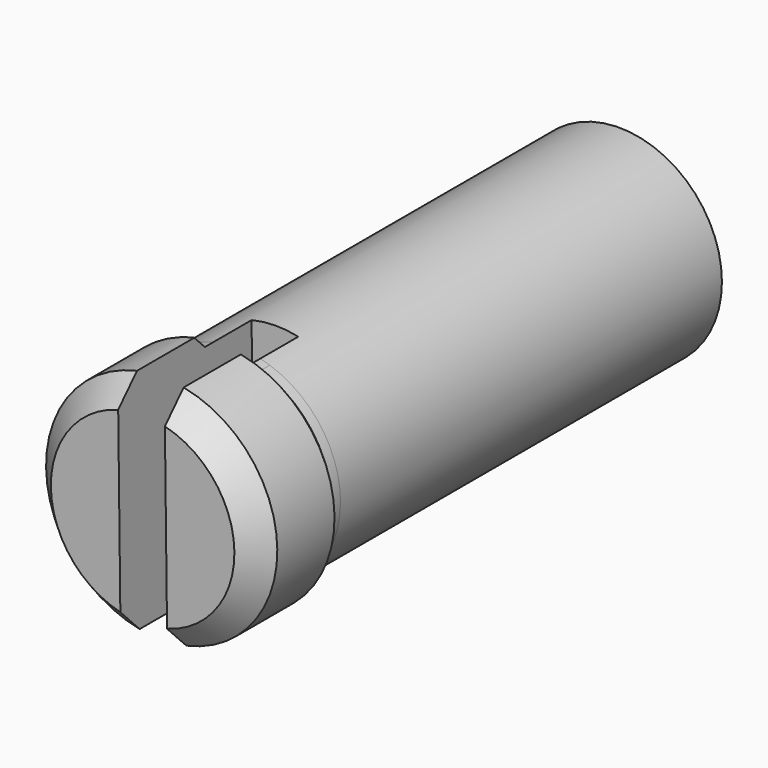
from build123d import *

# Parameters (mm, degrees)
F0_R         = 48.5
F0_R_2       = 43
F1_DEPTH     = 250
F2_DEPTH     = 200
F4_DEPTH     = 70
F5_T2_ANGLE  = 217.5315587112
F5_T4_ANGLE  = 217.5315587112
F5_T8_ANGLE  = 217.5315587112
F5_S9_R      = 43
F5_T10_DEPTH = 60
F5_T14_ANGLE = 217.5315587112
F5_S15_R     = 43
F5_T16_DEPTH = 60


# Not quite as in the source:
# - a fillet or chamfer that OpenCascade refuses, or shapes differently, is made with other operations: its cross-section is extruded or revolved along the edge and cut away or added


with BuildPart() as f1:
    # F0 (on Front) → F1 (new body)
    with BuildSketch(Plane.XZ):
        Circle(F0_R)
        Circle(F0_R_2, mode=Mode.SUBTRACT)
        Circle(F0_R_2)
    extrude(amount=F1_DEPTH)

    # F0 (on Front) → F2 (cut)
    with BuildSketch(Plane.XZ):
        Circle(F0_R)
        Circle(F0_R_2, mode=Mode.SUBTRACT)
    extrude(amount=F2_DEPTH, mode=Mode.SUBTRACT)

    # F3 (on face) → F4 (cut)
    with BuildSketch(Plane.XZ.offset(250)):
        with BuildLine():
            Line((10.3677597397, -47.3788935918), (9.2215594636, 47.6152584899))
            ThreePointArc((9.2215594636, 47.6152584899), (-0.5851588327, 48.4964698627), (-10.3677597397, 47.3788935918))
            Line((-10.3677597397, 47.3788935918), (-9.2215594636, -47.6152584899))
            ThreePointArc((-9.2215594636, -47.6152584899), (0.5851588327, -48.4964698627), (10.3677597397, -47.3788935918))
        make_face()
    extrude(amount=-F4_DEPTH, mode=Mode.SUBTRACT)

    # F5: chamfer of 10 on 4 edges, made by hand

    # F5_s1 → F5_t2 (revolve, cut)
    with BuildSketch(Plane(origin=(0, 0, 0), x_dir=(0, 1, 0), z_dir=(0.9506540069, 0, -0.3102530567))):
        Polygon((-240, 48.5), (-250, 38.5), (-250, 48.5), align=None)
    revolve(axis=Axis((0, -250, 0), (0, -1, 0)), revolution_arc=F5_T2_ANGLE, mode=Mode.SUBTRACT)

    # F5_s3 → F5_t4 (revolve, cut)
    with BuildSketch(Plane(origin=(0, 0, 0), x_dir=(0, 1, 0), z_dir=(-0.9428912961, 0, -0.3331005911))):
        Polygon((-240, -48.5), (-250, -38.5), (-250, -48.5), align=None)
    revolve(axis=Axis((0, -250, 0), (0, 1, 0)), revolution_arc=F5_T4_ANGLE, mode=Mode.SUBTRACT)


with BuildPart() as f5_tool6:
    # F5_s7 → F5_t8 (revolve)
    with BuildSketch(Plane(origin=(0, 0, 0), x_dir=(0, 1, 0), z_dir=(-0.9506540069, 0, 0.3102530567))):
        Polygon((-210, 48.5), (-200, 38.5), (-200, 48.5), align=None)
    revolve(axis=Axis((0, -200, 0), (0, -1, 0)), revolution_arc=F5_T8_ANGLE)

    # F5_s9 → F5_t10 (cut, symmetric)
    with BuildSketch(Plane.XZ.offset(205)):
        Circle(F5_S9_R)
    extrude(amount=F5_T10_DEPTH, both=True, mode=Mode.SUBTRACT)


with BuildPart() as f1_1:
    add(f1.part)

    # F5_t5: cut F5_tool6
    add(f5_tool6.part, mode=Mode.SUBTRACT)


with BuildPart() as f5_tool12:
    # F5_s13 → F5_t14 (revolve)
    with BuildSketch(Plane(origin=(0, 0, 0), x_dir=(0, 1, 0), z_dir=(0.9506540069, 0, -0.3102530567))):
        Polygon((-200, 38.5), (-210, 48.5), (-200, 48.5), align=None)
    revolve(axis=Axis((0, -200, 0), (0, -1, 0)), revolution_arc=F5_T14_ANGLE)

    # F5_s15 → F5_t16 (cut, symmetric)
    with BuildSketch(Plane.XZ.offset(205)):
        Circle(F5_S15_R)
    extrude(amount=F5_T16_DEPTH, both=True, mode=Mode.SUBTRACT)


with BuildPart() as f1_2:
    add(f1_1.part)

    # F5_t11: cut F5_tool12
    add(f5_tool12.part, mode=Mode.SUBTRACT)


solid = f1_2.part
